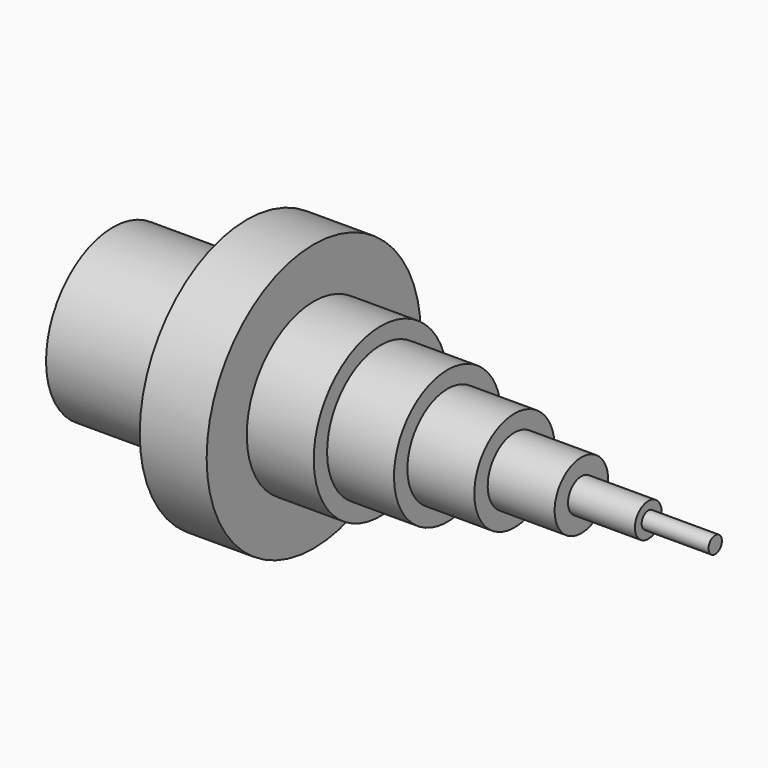
from build123d import *


# Not quite as in the source:
# - the program builds the solid bodies; features that only make, move or delete a surface that nothing else refers to are left out


with BuildPart() as f1:
    # F0 (on Front) → F1 (revolve)
    with BuildSketch(Plane.XZ):
        Polygon((-45.8035738753, 25), (-45.8035738753, 20), (-5.8035738753, 20), (-5.8035738753, 0), (134.1964261247, 0), (134.1964261247, 2.5), (114.1964261247, 2.5), (114.1964261247, 5), (94.1964261247, 5), (94.1964261247, 10), (74.1964261247, 10), (74.1964261247, 15), (54.1964261247, 15), (54.1964261247, 20), (34.1964261247, 20), (34.1964261247, 25), (14.1964261247, 25), (14.1964261247, 40), (-5.8035738753, 40), (-5.8035738753, 25), align=None)
    revolve(axis=Axis((44.1964261247, 0, 0), (-1, 0, 0)))


solid = f1.part
